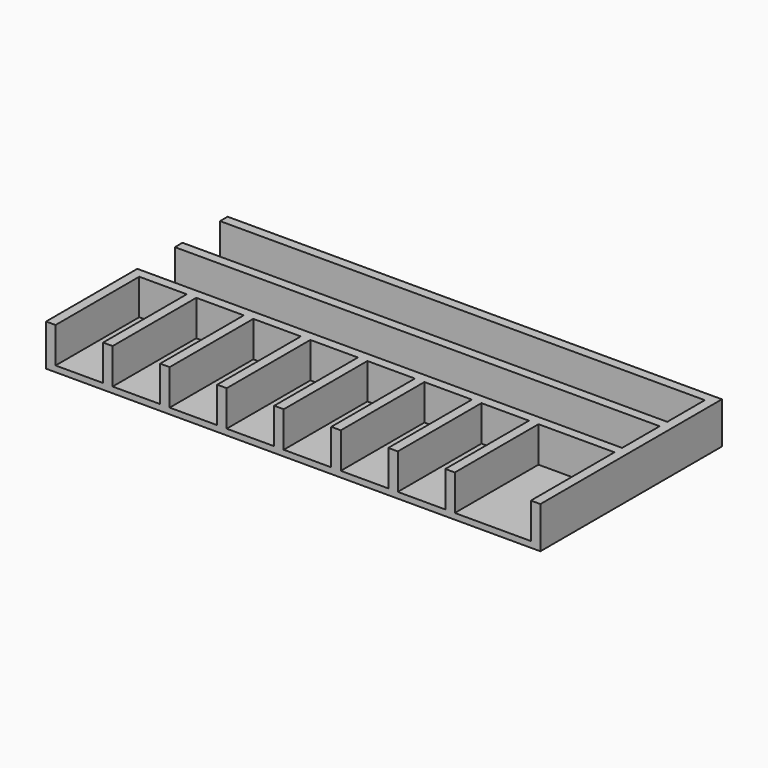
from build123d import *

# Parameters (mm, degrees)
F0_W     = 254
F0_H     = 25.0825
F1_DEPTH = 3.175
F2_DEPTH = 22.225
F3_DEPTH = 25.4


# Not quite as in the source:
# - a feature names something its author has since deleted; it is built from what else it names


with BuildPart() as f1:
    # F0 (on Top) → F1 (new body)
    with BuildSketch(Plane.XY):
        with Locations((-10.5066807906, 37.553641122)):
            Rectangle(F0_W, F0_H)
    extrude(amount=F1_DEPTH)



with BuildPart() as f1b:
    # F0 (on Top) → F1, piece 2 (new body)
    with BuildSketch(Plane.XY):
        with Locations((-10.5066807906, 7.391141122)):
            Rectangle(F0_W, F0_H)
    extrude(amount=F1_DEPTH)


with BuildPart() as f1c:
    # F0 (on Top) → F1, piece 3 (new body)
    with BuildSketch(Plane.XY):
        Polygon((-137.5066807906, -61.030108878), (-137.5066807906, -66.110108878), (-112.1066807906, -66.110108878), (-112.1066807906, -61.030108878), (-112.1066807906, -10.230108878), (-137.5066807906, -10.230108878), align=None)
    extrude(amount=F1_DEPTH)


with BuildPart() as f1d:
    # F0 (on Top) → F1, piece 4 (new body)
    with BuildSketch(Plane.XY):
        Polygon((-107.0266807906, -61.030108878), (-107.0266807906, -66.110108878), (-81.6266807906, -66.110108878), (-81.6266807906, -61.030108878), (-81.6266807906, -10.230108878), (-107.0266807906, -10.230108878), align=None)
    extrude(amount=F1_DEPTH)


with BuildPart() as f1e:
    # F0 (on Top) → F1, piece 5 (new body)
    with BuildSketch(Plane.XY):
        Polygon((-76.5466807906, -61.030108878), (-76.5466807906, -66.110108878), (-51.1466807906, -66.110108878), (-51.1466807906, -61.030108878), (-51.1466807906, -10.230108878), (-76.5466807906, -10.230108878), align=None)
    extrude(amount=F1_DEPTH)


with BuildPart() as f1f:
    # F0 (on Top) → F1, piece 6 (new body)
    with BuildSketch(Plane.XY):
        Polygon((-46.0666807906, -61.030108878), (-46.0666807906, -66.110108878), (-20.6666807906, -66.110108878), (-20.6666807906, -61.030108878), (-20.6666807906, -10.230108878), (-46.0666807906, -10.230108878), align=None)
    extrude(amount=F1_DEPTH)


with BuildPart() as f1g:
    # F0 (on Top) → F1, piece 7 (new body)
    with BuildSketch(Plane.XY):
        Polygon((-15.5866807906, -66.110108878), (9.8133192094, -66.110108878), (9.8133192094, -61.030108878), (9.8133192094, -10.230108878), (-15.5866807906, -10.230108878), (-15.5866807906, -61.030108878), align=None)
    extrude(amount=F1_DEPTH)


with BuildPart() as f1h:
    # F0 (on Top) → F1, piece 8 (new body)
    with BuildSketch(Plane.XY):
        Polygon((14.8933192094, -66.110108878), (40.2933192094, -66.110108878), (40.2933192094, -61.030108878), (40.2933192094, -10.230108878), (14.8933192094, -10.230108878), (14.8933192094, -61.030108878), align=None)
    extrude(amount=F1_DEPTH)


with BuildPart() as f1i:
    # F0 (on Top) → F1, piece 9 (new body)
    with BuildSketch(Plane.XY):
        Polygon((45.3733192094, -66.110108878), (70.7733192094, -66.110108878), (70.7733192094, -61.030108878), (70.7733192094, -10.230108878), (45.3733192094, -10.230108878), (45.3733192094, -61.030108878), align=None)
    extrude(amount=F1_DEPTH)


with BuildPart() as f1j:
    # F0 (on Top) → F1, piece 10 (new body)
    with BuildSketch(Plane.XY):
        Polygon((75.8533192094, -66.110108878), (116.4933192094, -66.110108878), (116.4933192094, -61.030108878), (116.4933192094, -10.230108878), (75.8533192094, -10.230108878), (75.8533192094, -61.030108878), align=None)
    extrude(amount=F1_DEPTH)


with BuildPart() as f1_1:
    add(f1.part)

    add(f1b.part)  # F2 merges F1b

    add(f1c.part)  # F2 merges F1c

    add(f1d.part)  # F2 merges F1d

    add(f1e.part)  # F2 merges F1e

    add(f1f.part)  # F2 merges F1f

    add(f1g.part)  # F2 merges F1g

    add(f1h.part)  # F2 merges F1h

    add(f1i.part)  # F2 merges F1i

    add(f1j.part)  # F2 merges F1j
    # F0 (on Top) → F2 (join)
    with BuildSketch(Plane.XY):
        Polygon((121.5733192094, 55.174891122), (-142.5866807906, 55.174891122), (-142.5866807906, -66.110108878), (-137.5066807906, -66.110108878), (-137.5066807906, -61.030108878), (-137.5066807906, -10.230108878), (-112.1066807906, -10.230108878), (-107.0266807906, -10.230108878), (-81.6266807906, -10.230108878), (-76.5466807906, -10.230108878), (-51.1466807906, -10.230108878), (-46.0666807906, -10.230108878), (-20.6666807906, -10.230108878), (-15.5866807906, -10.230108878), (9.8133192094, -10.230108878), (14.8933192094, -10.230108878), (40.2933192094, -10.230108878), (45.3733192094, -10.230108878), (70.7733192094, -10.230108878), (75.8533192094, -10.230108878), (116.4933192094, -10.230108878), (116.4933192094, -61.030108878), (116.4933192094, -66.110108878), (121.5733192094, -66.110108878), align=None)
        with Locations((-10.5066807906, 7.391141122)):
            Rectangle(F0_W, F0_H, mode=Mode.SUBTRACT)
        with Locations((-10.5066807906, 37.553641122)):
            Rectangle(F0_W, F0_H, mode=Mode.SUBTRACT)
        Polygon((-112.1066807906, -61.030108878), (-112.1066807906, -66.110108878), (-107.0266807906, -66.110108878), (-107.0266807906, -61.030108878), (-107.0266807906, -10.230108878), (-112.1066807906, -10.230108878), align=None)
        Polygon((-81.6266807906, -61.030108878), (-81.6266807906, -66.110108878), (-76.5466807906, -66.110108878), (-76.5466807906, -61.030108878), (-76.5466807906, -10.230108878), (-81.6266807906, -10.230108878), align=None)
        Polygon((-51.1466807906, -61.030108878), (-51.1466807906, -66.110108878), (-46.0666807906, -66.110108878), (-46.0666807906, -61.030108878), (-46.0666807906, -10.230108878), (-51.1466807906, -10.230108878), align=None)
        Polygon((-20.6666807906, -61.030108878), (-20.6666807906, -66.110108878), (-15.5866807906, -66.110108878), (-15.5866807906, -61.030108878), (-15.5866807906, -10.230108878), (-20.6666807906, -10.230108878), align=None)
        Polygon((9.8133192094, -66.110108878), (14.8933192094, -66.110108878), (14.8933192094, -61.030108878), (14.8933192094, -10.230108878), (9.8133192094, -10.230108878), (9.8133192094, -61.030108878), align=None)
        Polygon((40.2933192094, -66.110108878), (45.3733192094, -66.110108878), (45.3733192094, -61.030108878), (45.3733192094, -10.230108878), (40.2933192094, -10.230108878), (40.2933192094, -61.030108878), align=None)
        Polygon((70.7733192094, -66.110108878), (75.8533192094, -66.110108878), (75.8533192094, -61.030108878), (75.8533192094, -10.230108878), (70.7733192094, -10.230108878), (70.7733192094, -61.030108878), align=None)
    extrude(amount=F2_DEPTH)

    # F3 (cut): faces of the model
    f3_faces = [f1_1.faces().sort_by_distance(p)[0] for p in [
        (-137.5066807906, 7.391141122, 12.7),
        (-137.5066807906, 37.553641122, 12.7),
    ]]
    extrude(f3_faces, amount=-F3_DEPTH, mode=Mode.SUBTRACT)


solid = f1_1.part
